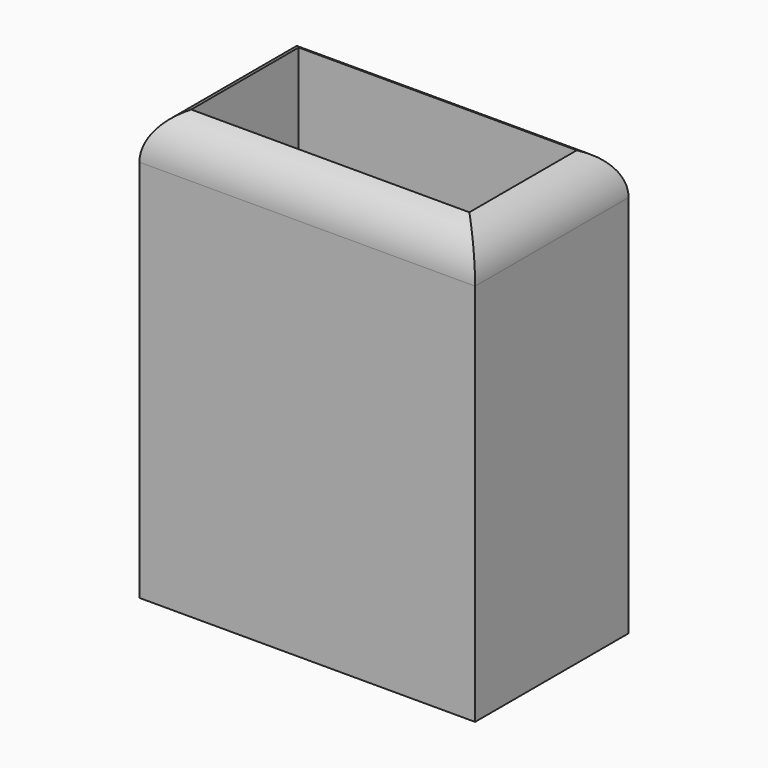
from build123d import *

# Parameters (mm, degrees)
F0_W        = 35
F0_H        = 20
F1_DEPTH    = 45
F2_W        = 29
F2_H        = 14
F3_DEPTH    = 40
F4_T1_DEPTH = 60
F4_T3_DEPTH = 45


# Not quite as in the source:
# - a fillet or chamfer that OpenCascade refuses, or shapes differently, is made with other operations: its cross-section is extruded or revolved along the edge and cut away or added


with BuildPart() as f1:
    # F0 (on Top) → F1 (new body)
    with BuildSketch(Plane.XY):
        Rectangle(F0_W, F0_H)
    extrude(amount=F1_DEPTH)

    # F2 (on face) → F3 (cut)
    with BuildSketch(Plane.XY.offset(45)):
        Rectangle(F2_W, F2_H)
    extrude(amount=-F3_DEPTH, mode=Mode.SUBTRACT)

    # F4: fillet of radius 5 on 4 edges, made by hand

    # F4_s2 → F4_t1 (cut)
    with BuildSketch(Plane.YZ.offset(-30)):
        with BuildLine():
            ThreePointArc((-10, 40), (-8.5355339059, 43.5355339059), (-5, 45))
            Line((-5, 45), (-10, 45))
            Line((-10, 45), (-10, 40))
        make_face()
        with BuildLine():
            ThreePointArc((5, 45), (8.5355339059, 43.5355339059), (10, 40))
            Line((10, 40), (10, 45))
            Line((10, 45), (5, 45))
        make_face()
    extrude(amount=F4_T1_DEPTH, mode=Mode.SUBTRACT)

    # F4_s4 → F4_t3 (cut)
    with BuildSketch(Plane.XZ.offset(-22.5)):
        with BuildLine():
            ThreePointArc((-17.5, 40), (-16.0355339059, 43.5355339059), (-12.5, 45))
            Line((-12.5, 45), (-17.5, 45))
            Line((-17.5, 45), (-17.5, 40))
        make_face()
        with BuildLine():
            ThreePointArc((17.5, 40), (16.0355339059, 43.5355339059), (12.5, 45))
            Line((12.5, 45), (17.5, 45))
            Line((17.5, 45), (17.5, 40))
        make_face()
    extrude(amount=F4_T3_DEPTH, mode=Mode.SUBTRACT)


solid = f1.part
